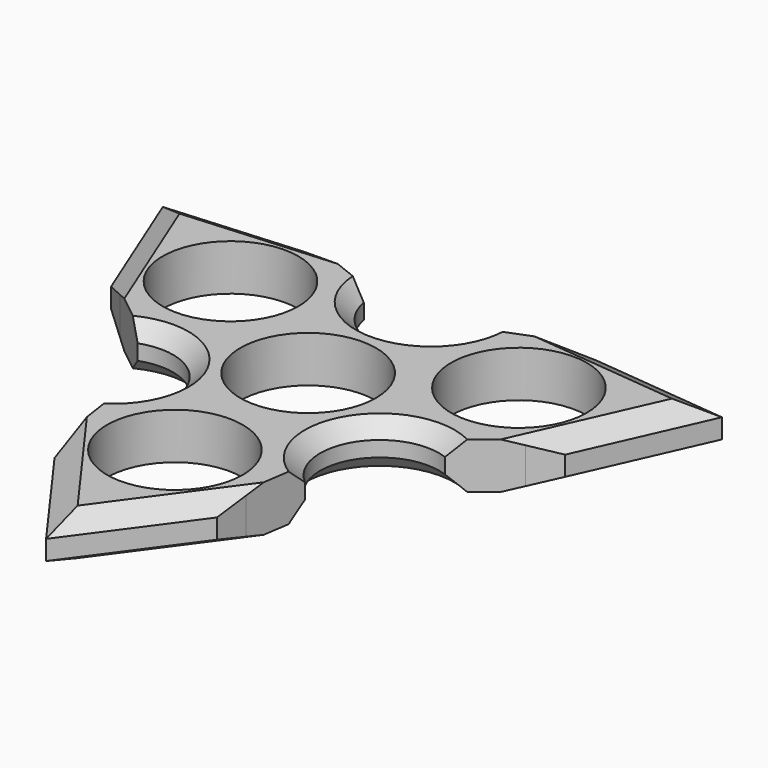
from build123d import *

# Parameters (mm, degrees)
F0_R       = 11.176
F1_DEPTH   = 7.62
F2_SIZE2   = 2.1997045256
F2_SIZE    = 3.81
F2_2_SIZE2 = 2.1997045256
F2_2_SIZE  = 3.81
F3_SIZE2   = 2.1997045256
F3_SIZE    = 3.81
F4_SIZE    = 2.54


# Not quite as in the source:
# - a feature names something its author has since deleted; it is built from what else it names


with BuildPart() as f1:
    # F0 (on Top) → F1 (new body)
    with BuildSketch(Plane.XY):
        with BuildLine():
            ThreePointArc((9.7057271537, 23.5283748909), (-0.0208649872, 15.4470615517), (-9.6943160077, 23.5919105566))
            Line((-9.6943160077, 23.5919105566), (-19.3886320155, 27.4654462223))
            Line((-19.3886320155, 27.4654462223), (-24.1059964708, 29.3503527439))
            Line((-24.1059964708, 29.3503527439), (-46.1373193312, 27.748740566))
            Line((-46.1373193312, 27.748740566), (-37.463364806, 6.2451757293))
            Line((-37.463364806, 6.2451757293), (-33.4914395336, 3.0781251091))
            Line((-33.4914395336, 3.0781251091), (-25.3390191684, -3.4222811682))
            ThreePointArc((-25.3390191684, -3.4222811682), (-13.4326493579, -7.7553437227), (-15.6332920147, -20.2330937227))
            Line((-15.6332920147, -20.2330937227), (-14.0799852263, -30.5435))
            Line((-14.0799852263, -30.5435), (-13.3232015704, -35.5668134979))
            Line((-13.3232015704, -35.5668134979), (-0.0898891733, -53.8478470607))
            Line((-0.0898891733, -53.8478470607), (13.3370282377, -35.4750360336))
            Line((13.3370282377, -35.4750360336), (14.0938118937, -30.4517225357))
            Line((14.0938118937, -30.4517225357), (15.6402053484, -20.1872049906))
            ThreePointArc((15.6402053484, -20.1872049906), (13.4326493579, -7.7553437227), (25.3027350274, -3.4512126568))
            Line((25.3027350274, -3.4512126568), (33.4188712518, 3.0202621318))
            Line((33.4188712518, 3.0202621318), (37.3907965242, 6.1873127519))
            Line((37.3907965242, 6.1873127519), (46.633735943, 26.924))
            Line((46.633735943, 26.924), (24.1401632357, 29.1946377686))
            Line((24.1401632357, 29.1946377686), (19.4114543073, 27.3383748909))
            Line((19.4114543073, 27.3383748909), (9.7057271537, 23.5283748909))
        make_face()
        with Locations((0, -27.432)):
            Circle(F0_R, mode=Mode.SUBTRACT)
        Circle(F0_R, mode=Mode.SUBTRACT)
        with Locations((-23.7568088766, 13.716)):
            Circle(F0_R, mode=Mode.SUBTRACT)
        with Locations((23.7568088766, 13.716)):
            Circle(F0_R, mode=Mode.SUBTRACT)
    extrude(amount=F1_DEPTH)

    # F2
    f2_edges = [f1.edges().sort_by_distance(p)[0] for p in [
        (-41.800342, 16.996958, 7.62),
        (-35.121658, 28.549547, 7.62),
        (35.38695, 28.059319, 7.62),
        (42.012266, 16.555656, 7.62),
        (6.62357, -44.661442, 7.62),
        (-6.706545, -44.70733, 7.62),
    ]]
    f2_side = f1.faces().sort_by_distance((13.256392, -27.645481, 7.62))[0]
    chamfer(f2_edges, length=F2_SIZE, length2=F2_SIZE2, reference=f2_side)

    # F2#2
    f2_2_edges = [f1.edges().sort_by_distance(p)[0] for p in [
        (-41.800342, 16.996958, 0),
        (42.012266, 16.555656, 0),
        (-35.121658, 28.549547, 0),
    ]]
    f2_2_side = f1.faces().sort_by_distance((12.353469, -7.132279, 0))[0]
    chamfer(f2_2_edges, length=F2_2_SIZE, length2=F2_2_SIZE2, reference=f2_2_side)

    # F3
    f3_edges = [f1.edges().sort_by_distance(p)[0] for p in [
        (-6.706545, -44.70733, 0),
        (6.62357, -44.661442, 0),
        (33.391083, 28.260794, 0),
    ]]
    f3_side = f1.faces().sort_by_distance((27.377875, -0.292303, 0))[0]
    chamfer(f3_edges, length=F3_SIZE, length2=F3_SIZE2, reference=f3_side)

    # F4
    f4_edges = [f1.edges().sort_by_distance(p)[0] for p in [
        (-0.020865, 15.447062, 7.62),
        (13.432649, -7.755344, 7.62),
        (-13.432649, -7.755344, 7.62),
        (-13.432649, -7.755344, 0),
        (-0.020865, 15.447062, 0),
        (13.432649, -7.755344, 0),
    ]]
    chamfer(f4_edges, length=F4_SIZE)


solid = f1.part
